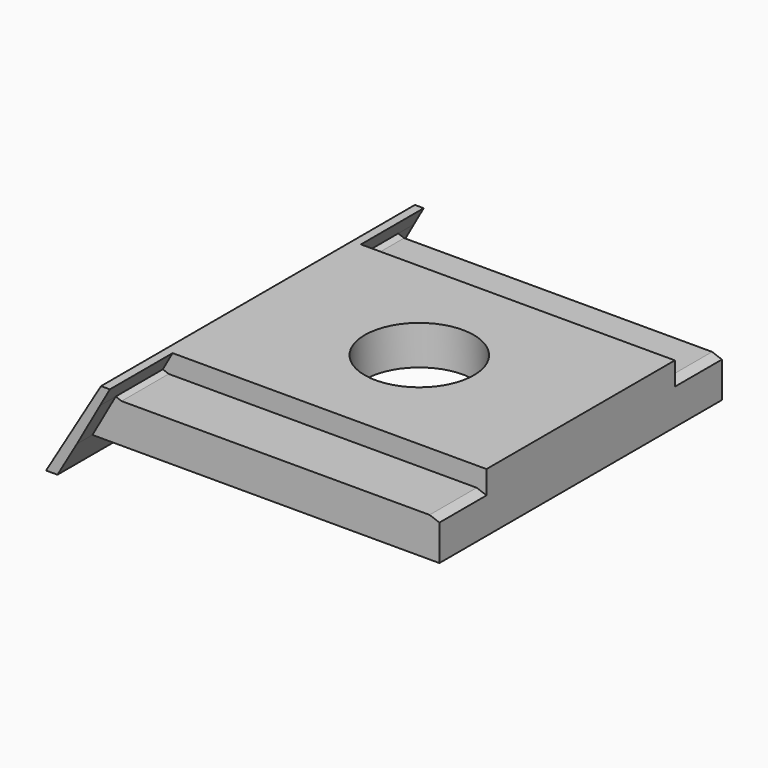
from build123d import *

# Parameters (mm, degrees)
F1_DEPTH  = 20
F3_DEPTH  = 4
F5_DEPTH  = 1
F7_DEPTH  = 20.001
F10_W     = 15
F10_H     = 9.1
F11_DEPTH = 1
F12_D     = 5.55752


# Not quite as in the source:
# - a pattern or mirror of a feature is missing from the dataset's text; its kind, count and spacing are read off the source's solid


with BuildPart() as f1:
    # F0 (on Front) → F1 (new body)
    with BuildSketch(Plane.XZ):
        Polygon((-16.45, 3), (-19.25, -1.7), (-18.09, -1.7), (-17.0772340426, 0), (0, 0), (0, 3), align=None)
    extrude(amount=F1_DEPTH)

    # F2 (on face) → F3 (cut)
    with BuildSketch(Plane.XZ.offset(20)):
        Polygon((-16.2, 2), (-0.5, 2), (0, 1.8180148829), (0, 3), (-16, 3), (-16.5, 2.1091910703), align=None)
    f3 = extrude(amount=-F3_DEPTH, mode=Mode.SUBTRACT)

    # F3_copies: F3 across plane
    add(f3.mirror(Plane.ZX.offset(-10)), mode=Mode.SUBTRACT)

    # F4 (on face) → F5 (cut)
    with BuildSketch(Plane.XZ.offset(20)):
        Polygon((0, 0), (0, 1.8180148829), (-0.5, 2), (-16.2, 2), (-16.5, 2.1091910703), (-17.683862779, 0), align=None)
    f5 = extrude(amount=-F5_DEPTH, mode=Mode.SUBTRACT)

    # F5_copies: F5 across plane
    add(f5.mirror(Plane.ZX.offset(-10)), mode=Mode.SUBTRACT)

    # F6 (on face) → F7 (cut, through all)
    with BuildSketch(Plane.XZ.offset(20)):
        Polygon((-18.67, -1.7), (-18.09, -1.7), (-17.0772340426, 0), (-17.683862779, 0), align=None)
    extrude(amount=-F7_DEPTH, mode=Mode.SUBTRACT)

    # F10 (on face) → F11 (cut)
    with BuildSketch(Plane(origin=(0, 0, 0), x_dir=(1, 0, 0), z_dir=(0, 0, -1))):
        with Locations((-9, 10)):
            Rectangle(F10_W, F10_H)
    extrude(amount=-F11_DEPTH, mode=Mode.SUBTRACT)

    # F12 (through all)
    with Locations(Plane.XY.offset(3)):
        with Locations((-8.225, -10)):
            Hole(F12_D / 2)


solid = f1.part
